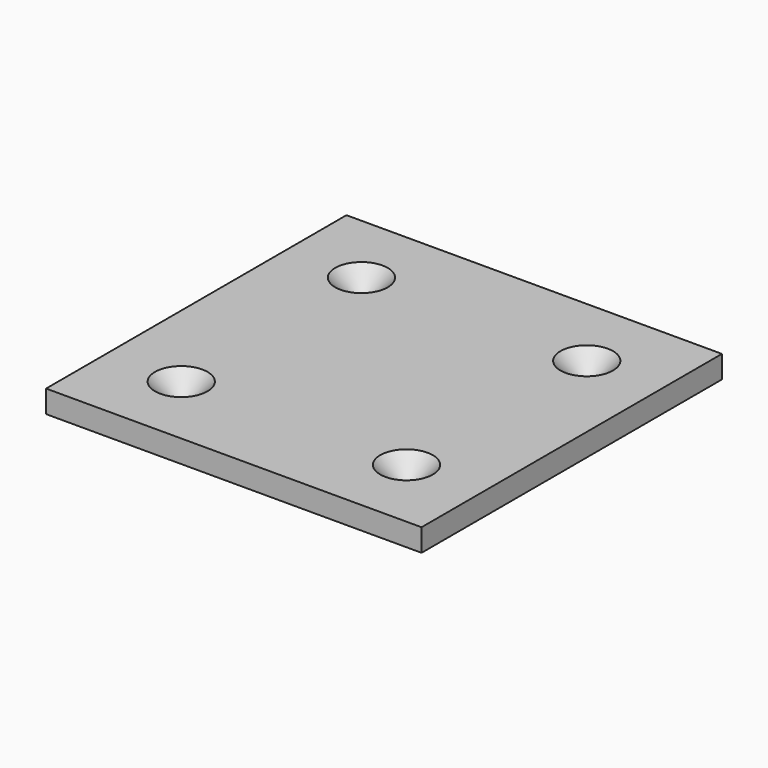
from build123d import *

# Parameters (mm, degrees)
F0_W     = 40
F0_H     = 40
F0_R     = 0.3
F1_DEPTH = 2.4


# Not quite as in the source:
# - a fillet or chamfer that OpenCascade refuses, or shapes differently, is made with other operations: its cross-section is extruded or revolved along the edge and cut away or added


with BuildPart() as f1:
    # F0 (on Top) → F1 (new body)
    with BuildSketch(Plane.XY):
        Rectangle(F0_W, F0_H)
        with Locations((-12, -12)):
            Circle(F0_R, mode=Mode.SUBTRACT)
        with Locations((12, -12)):
            Circle(F0_R, mode=Mode.SUBTRACT)
        with Locations((-12, 12)):
            Circle(F0_R, mode=Mode.SUBTRACT)
        with Locations((12, 12)):
            Circle(F0_R, mode=Mode.SUBTRACT)
    extrude(amount=F1_DEPTH)

    # F2: chamfer of 2.5 on 4 edges, made by hand

    # F2_s1 → F2_t2 (revolve, cut)
    with BuildSketch(Plane.XZ.offset(-12)):
        Polygon((-11.7, -0.1), (-9.2, 2.4), (-11.7, 2.4), align=None)
    revolve(axis=Axis((-12, 12, 2.4), (0, 0, 1)), mode=Mode.SUBTRACT)

    # F2_s3 → F2_t4 (revolve, cut)
    with BuildSketch(Plane.XZ.offset(-12)):
        Polygon((12.3, -0.1), (14.8, 2.4), (12.3, 2.4), align=None)
    revolve(axis=Axis((12, 12, 2.4), (0, 0, 1)), mode=Mode.SUBTRACT)

    # F2_s5 → F2_t6 (revolve, cut)
    with BuildSketch(Plane.XZ.offset(12)):
        Polygon((12.3, -0.1), (14.8, 2.4), (12.3, 2.4), align=None)
    revolve(axis=Axis((12, -12, 2.4), (0, 0, 1)), mode=Mode.SUBTRACT)

    # F2_s7 → F2_t8 (revolve, cut)
    with BuildSketch(Plane.XZ.offset(12)):
        Polygon((-11.7, -0.1), (-9.2, 2.4), (-11.7, 2.4), align=None)
    revolve(axis=Axis((-12, -12, 2.4), (0, 0, 1)), mode=Mode.SUBTRACT)


solid = f1.part
